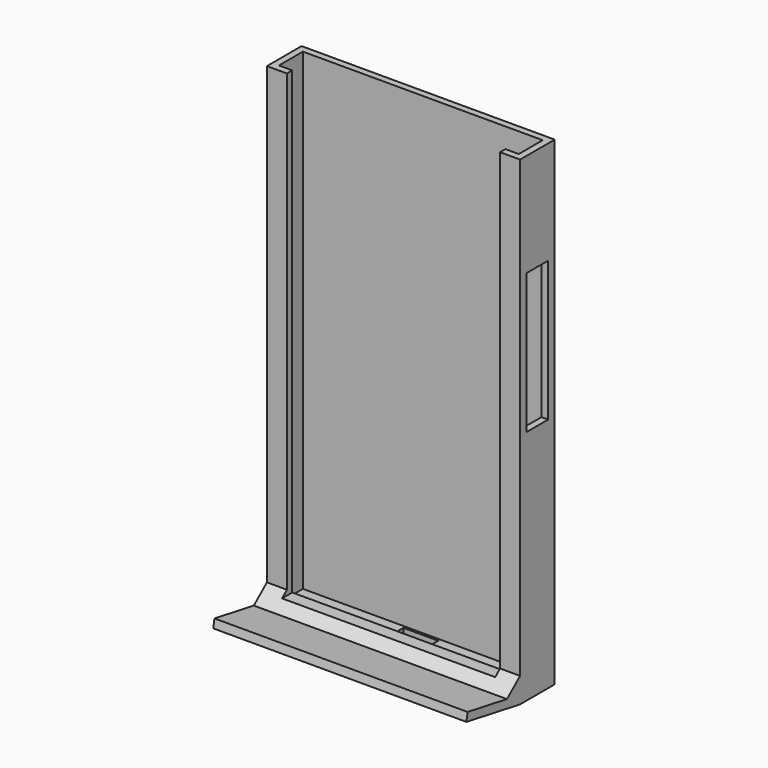
from build123d import *

# Parameters (mm, degrees)
F0_W          = 76
F0_H          = 144
F1_DEPTH      = 13
F3_DEPTH      = 142
F4_W          = 64
F4_H          = 2
F5_DEPTH      = 4
F6_W          = 10.5
F6_H          = 7.5
F7_DEPTH      = 25
F8_W          = 8.0420786627
F8_H          = 42
F9_DEPTH      = 25
F11_DEPTH     = 76
F12_T4_DEPTH  = 76
F12_T10_DEPTH = 76
F12_T16_DEPTH = 76
F12_T23_DEPTH = 76
F12_T29_DEPTH = 76


# Not quite as in the source:
# - a fillet or chamfer that OpenCascade refuses, or shapes differently, is made with other operations: its cross-section is extruded or revolved along the edge and cut away or added


with BuildPart() as f1:
    # F0 (on Front) → F1 (new body)
    with BuildSketch(Plane.XZ):
        Rectangle(F0_W, F0_H)
    extrude(amount=F1_DEPTH)

    # F2 (on face) → F3 (cut)
    with BuildSketch(Plane.XY.offset(72)):
        Polygon((-32, -11), (-32, -13), (32, -13), (32, -11), (36, -11), (36, -2), (-36, -2), (-36, -11), align=None)
    extrude(amount=-F3_DEPTH, mode=Mode.SUBTRACT)

    # F4 (on face) → F5 (join)
    with BuildSketch(Plane.XY.offset(-70)):
        with Locations((0, -12)):
            Rectangle(F4_W, F4_H)
    extrude(amount=F5_DEPTH)

    # F6 (on face) → F7 (cut)
    with BuildSketch(Plane(origin=(0, 0, -72), x_dir=(1, 0, 0), z_dir=(0, 0, -1))):
        with Locations((0, 6.5)):
            Rectangle(F6_W, F6_H)
    extrude(amount=-F7_DEPTH, mode=Mode.SUBTRACT)

    # F8 (on face) → F9 (cut)
    with BuildSketch(Plane.YZ.offset(38)):
        with Locations((-6.5, 20)):
            Rectangle(F8_W, F8_H)
    extrude(amount=-F9_DEPTH, mode=Mode.SUBTRACT)

    # F10 (on face) → F11 (join)
    with BuildSketch(Plane.YZ.offset(38)):
        Polygon((-33.1302755044, -68.4504892995), (-13, -72), (-13, -69.4614334703), (-32.6961550602, -65.9884699169), align=None)
    extrude(amount=-F11_DEPTH)

    # F12: chamfer of 5 on 1 edges, made by hand


with BuildPart() as f12_tool2:
    # F12_s3 → F12_t4 (new body)
    with BuildSketch(Plane.YZ.offset(38)):
        Polygon((-13, -64.4614334703), (-17.9240387651, -68.593192582), (-13, -69.4614334703), align=None)
    extrude(amount=-F12_T4_DEPTH)

    split(bisect_by=Plane.XY.offset(-66), keep=Keep.TOP)

    split(bisect_by=Plane.YZ.offset(32), keep=Keep.TOP)


with BuildPart() as f1_1:
    add(f1.part)

    # F12_t1: union F12_tool2
    add(f12_tool2.part)


with BuildPart() as f12_tool8:
    # F12_s9 → F12_t10 (new body)
    with BuildSketch(Plane.YZ.offset(38)):
        Polygon((-13, -64.4614334703), (-17.9240387651, -68.593192582), (-13, -69.4614334703), align=None)
    extrude(amount=-F12_T10_DEPTH)

    split(bisect_by=Plane.XY.offset(-66), keep=Keep.BOTTOM)

    split(bisect_by=Plane.YZ.offset(32), keep=Keep.TOP)


with BuildPart() as f1_2:
    add(f1_1.part)

    # F12_t7: union F12_tool8
    add(f12_tool8.part)


with BuildPart() as f12_tool14:
    # F12_s15 → F12_t16 (new body)
    with BuildSketch(Plane.YZ.offset(38)):
        Polygon((-13, -64.4614334703), (-17.9240387651, -68.593192582), (-13, -69.4614334703), align=None)
    extrude(amount=-F12_T16_DEPTH)

    split(bisect_by=Plane.YZ.offset(-32), keep=Keep.TOP)

    split(bisect_by=Plane.XY.offset(-66), keep=Keep.BOTTOM)

    split(bisect_by=Plane.YZ.offset(32), keep=Keep.BOTTOM)


with BuildPart() as f1_3:
    add(f1_2.part)

    # F12_t13: union F12_tool14
    add(f12_tool14.part)


with BuildPart() as f12_tool21:
    # F12_s22 → F12_t23 (new body)
    with BuildSketch(Plane.YZ.offset(38)):
        Polygon((-13, -64.4614334703), (-17.9240387651, -68.593192582), (-13, -69.4614334703), align=None)
    extrude(amount=-F12_T23_DEPTH)

    split(bisect_by=Plane.YZ.offset(-32), keep=Keep.BOTTOM)

    split(bisect_by=Plane.XY.offset(-66), keep=Keep.TOP)


with BuildPart() as f1_4:
    add(f1_3.part)

    # F12_t20: union F12_tool21
    add(f12_tool21.part)


with BuildPart() as f12_tool27:
    # F12_s28 → F12_t29 (new body)
    with BuildSketch(Plane.YZ.offset(38)):
        Polygon((-13, -64.4614334703), (-17.9240387651, -68.593192582), (-13, -69.4614334703), align=None)
    extrude(amount=-F12_T29_DEPTH)

    split(bisect_by=Plane.YZ.offset(-32), keep=Keep.BOTTOM)

    split(bisect_by=Plane.XY.offset(-66), keep=Keep.BOTTOM)


with BuildPart() as f1_5:
    add(f1_4.part)

    # F12_t26: union F12_tool27
    add(f12_tool27.part)


solid = f1_5.part
